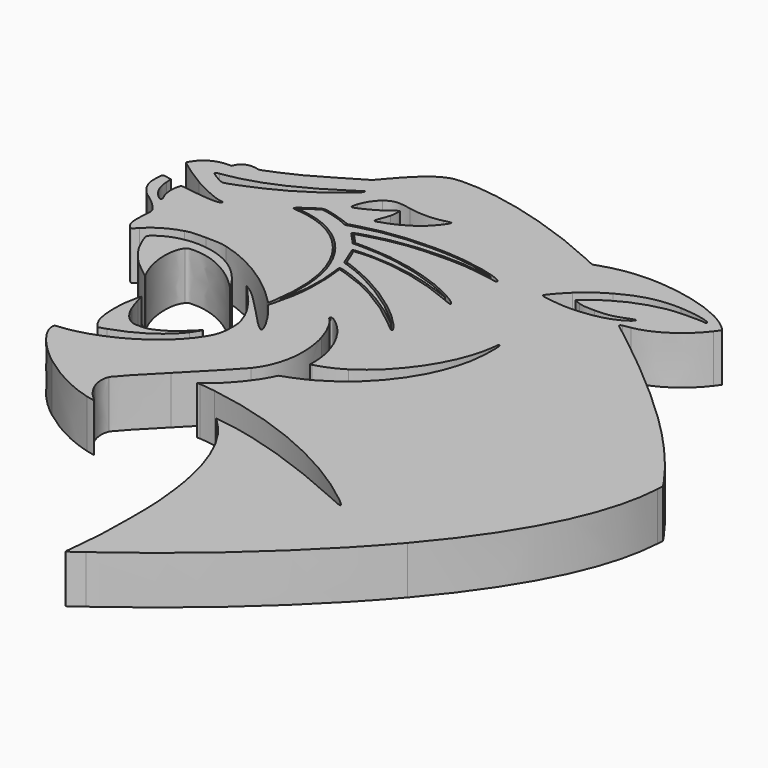
from build123d import *

# Parameters (mm, degrees)
F1_DEPTH = 10


# Not quite as in the source:
# - ends of sketch curves that miss each other by under 0.0002 mm in the source are joined


with BuildPart() as f1:
    # F0 (on Top) → F1 (new body)
    with BuildSketch(Plane.XY):
        with BuildLine():
            add(Edge.make_bspline(
                [(-23.607011, 20.41253), (-23.555899, 20.466755), (-23.36464, 21.326937), (-23.181995, 22.324017)],
                knots=[0, 0, 0, 0, 1, 1, 1, 1], degree=3))
            add(Edge.make_bspline(
                [(-23.181995, 22.324017), (-22.492284, 26.088964), (-22.389352, 30.089862), (-22.897956, 33.36236)],
                knots=[0, 0, 0, 0, 1, 1, 1, 1], degree=3))
            add(Edge.make_bspline(
                [(-22.897956, 33.36236), (-23.019357, 34.143477), (-23.068107, 34.840872), (-23.006291, 34.912122)],
                knots=[0, 0, 0, 0, 1, 1, 1, 1], degree=3))
            add(Edge.make_bspline(
                [(-23.006291, 34.912122), (-22.769167, 35.185415), (-18.48955, 33.680779), (-15.558898, 32.29376)],
                knots=[0, 0, 0, 0, 1, 1, 1, 1], degree=3))
            add(Edge.make_bspline(
                [(-15.558898, 32.29376), (-12.058682, 30.637175), (-7.348256, 27.560307), (-4.801806, 25.267182)],
                knots=[0, 0, 0, 0, 1, 1, 1, 1], degree=3))
            add(Edge.make_bspline(
                [(-4.801806, 25.267182), (-4.500624, 24.995967), (-4.300395, 24.860352), (-4.356852, 24.96584)],
                knots=[0, 0, 0, 0, 1, 1, 1, 1], degree=3))
            add(Edge.make_bspline(
                [(-4.356852, 24.96584), (-4.574715, 25.372872), (-7.364497, 27.840845), (-9.01195, 29.083962)],
                knots=[0, 0, 0, 0, 1, 1, 1, 1], degree=3))
            add(Edge.make_bspline(
                [(-9.01195, 29.083962), (-13.459709, 32.440107), (-18.866425, 35.386422), (-22.748893, 36.569729)],
                knots=[0, 0, 0, 0, 1, 1, 1, 1], degree=3))
            add(Edge.make_bspline(
                [(-22.748893, 36.569729), (-23.476911, 36.791617), (-23.718841, 36.937543), (-23.775043, 37.188685)],
                knots=[0, 0, 0, 0, 1, 1, 1, 1], degree=3))
            add(Edge.make_bspline(
                [(-23.775043, 37.188685), (-23.81549, 37.369424), (-24.179792, 38.281077), (-24.584599, 39.214579)],
                knots=[0, 0, 0, 0, 1, 1, 1, 1], degree=3))
            add(Edge.make_bspline(
                [(-24.584599, 39.214579), (-24.989408, 40.148082), (-25.320615, 40.980952), (-25.320615, 41.065402)],
                knots=[0, 0, 0, 0, 1, 1, 1, 1], degree=3))
            add(Edge.make_bspline(
                [(-25.320615, 41.065402), (-25.320615, 41.330584), (-24.374488, 41.416412), (-21.450763, 41.416462)],
                knots=[0, 0, 0, 0, 1, 1, 1, 1], degree=3))
            add(Edge.make_bspline(
                [(-21.450763, 41.416462), (-15.907912, 41.416555), (-10.712137, 40.427282), (-5.242939, 38.3305)],
                knots=[0, 0, 0, 0, 1, 1, 1, 1], degree=3))
            add(Edge.make_bspline(
                [(-5.242939, 38.3305), (-4.044155, 37.87091), (-3.111244, 37.541015), (-3.169804, 37.597399)],
                knots=[0, 0, 0, 0, 1, 1, 1, 1], degree=3))
            add(Edge.make_bspline(
                [(-3.169804, 37.597399), (-3.452747, 37.869826), (-5.755507, 38.953568), (-7.588494, 39.676957)],
                knots=[0, 0, 0, 0, 1, 1, 1, 1], degree=3))
            add(Edge.make_bspline(
                [(-7.588494, 39.676957), (-13.021844, 41.821228), (-19.037966, 43.012825), (-24.43056, 43.012825)],
                knots=[0, 0, 0, 0, 1, 1, 1, 1], degree=3))
            Line((-24.43056, 43.012825), (-26.740849, 43.012825))
            Line((-26.740849, 43.012825), (-27.585583, 43.951994))
            add(Edge.make_bspline(
                [(-27.585583, 43.951994), (-28.050187, 44.468535), (-28.6169, 45.072836), (-28.844945, 45.294882)],
                knots=[0, 0, 0, 0, 1, 1, 1, 1], degree=3))
            add(Edge.make_bspline(
                [(-28.844945, 45.294882), (-29.131999, 45.574386), (-29.215641, 45.750195), (-29.11679, 45.866281)],
                knots=[0, 0, 0, 0, 1, 1, 1, 1], degree=3))
            add(Edge.make_bspline(
                [(-29.11679, 45.866281), (-28.899874, 46.121018), (-24.878314, 47.26273), (-22.658669, 47.699727)],
                knots=[0, 0, 0, 0, 1, 1, 1, 1], degree=3))
            add(Edge.make_bspline(
                [(-22.658669, 47.699727), (-16.690853, 48.874652), (-10.13353, 49.022795), (-4.036425, 48.120442)],
                knots=[0, 0, 0, 0, 1, 1, 1, 1], degree=3))
            add(Edge.make_bspline(
                [(-4.036425, 48.120442), (-2.934208, 47.957317), (-2.012859, 47.845072), (-1.988982, 47.871005)],
                knots=[0, 0, 0, 0, 1, 1, 1, 1], degree=3))
            add(Edge.make_bspline(
                [(-1.988982, 47.871005), (-1.885069, 47.983876), (-5.101598, 48.762421), (-6.86971, 49.052363)],
                knots=[0, 0, 0, 0, 1, 1, 1, 1], degree=3))
            add(Edge.make_bspline(
                [(-6.86971, 49.052363), (-9.744468, 49.523776), (-12.162409, 49.703075), (-15.639058, 49.702643)],
                knots=[0, 0, 0, 0, 1, 1, 1, 1], degree=3))
            add(Edge.make_bspline(
                [(-15.639058, 49.702643), (-21.335491, 49.701981), (-25.526134, 49.145658), (-30.173319, 47.773322)],
                knots=[0, 0, 0, 0, 1, 1, 1, 1], degree=3))
            Line((-30.173319, 47.773322), (-31.778112, 47.299418))
            Line((-31.778112, 47.299418), (-32.799291, 47.76548))
            add(Edge.make_bspline(
                [(-32.799291, 47.76548), (-33.932578, 48.282708), (-35.678107, 48.809259), (-37.107958, 49.06522)],
                knots=[0, 0, 0, 0, 1, 1, 1, 1], degree=3))
            Line((-37.107958, 49.06522), (-38.045893, 49.233122))
            Line((-38.045893, 49.233122), (-39.730176, 48.074284))
            Line((-39.730176, 48.074284), (-41.414458, 46.915445))
            Line((-41.414458, 46.915445), (-40.865376, 46.87577))
            add(Edge.make_bspline(
                [(-40.865376, 46.87577), (-32.764973, 46.290472), (-26.281806, 40.581082), (-24.167065, 32.17043)],
                knots=[0, 0, 0, 0, 1, 1, 1, 1], degree=3))
            add(Edge.make_bspline(
                [(-24.167065, 32.17043), (-23.525104, 29.617257), (-23.341412, 27.648612), (-23.432327, 24.296187)],
                knots=[0, 0, 0, 0, 1, 1, 1, 1], degree=3))
            add(Edge.make_bspline(
                [(-23.432327, 24.296187), (-23.47747, 22.6316), (-23.556139, 21.054619), (-23.607149, 20.79179)],
                knots=[0, 0, 0, 0, 1, 1, 1, 1], degree=3))
            add(Edge.make_bspline(
                [(-23.607149, 20.79179), (-23.658157, 20.52896), (-23.658074, 20.358297), (-23.607011, 20.41253)],
                knots=[0, 0, 0, 0, 1, 1, 1, 1], degree=3))
        make_face()
    extrude(amount=F1_DEPTH)


with BuildPart() as f1b:
    # F0 (on Top) → F1, piece 2 (new body)
    with BuildSketch(Plane.XY):
        with BuildLine():
            add(Edge.make_bspline(
                [(4.705259, -70.782003), (4.800284, -70.717803), (5.966422, -69.878711), (7.296682, -68.917368)],
                knots=[0, 0, 0, 0, 1, 1, 1, 1], degree=3))
            add(Edge.make_bspline(
                [(7.296682, -68.917368), (21.832102, -58.413018), (35.938987, -45.615086), (46.067909, -33.743658)],
                knots=[0, 0, 0, 0, 1, 1, 1, 1], degree=3))
            add(Edge.make_bspline(
                [(46.067909, -33.743658), (58.546252, -19.118643), (65.216864, -5.670423), (65.968147, 6.375994)],
                knots=[0, 0, 0, 0, 1, 1, 1, 1], degree=3))
            Line((65.968147, 6.375994), (66.052589, 7.729962))
            Line((66.052589, 7.729962), (65.261452, 8.924637))
            add(Edge.make_bspline(
                [(65.261452, 8.924637), (62.172787, 13.588767), (56.377229, 20.249052), (50.267025, 26.156322)],
                knots=[0, 0, 0, 0, 1, 1, 1, 1], degree=3))
            add(Edge.make_bspline(
                [(50.267025, 26.156322), (44.572132, 31.662079), (36.743707, 38.382701), (28.749952, 44.628517)],
                knots=[0, 0, 0, 0, 1, 1, 1, 1], degree=3))
            add(Edge.make_bspline(
                [(28.749952, 44.628517), (26.946637, 46.03751), (25.393462, 47.225745), (25.298437, 47.269039)],
                knots=[0, 0, 0, 0, 1, 1, 1, 1], degree=3))
            add(Edge.make_bspline(
                [(25.298437, 47.269039), (24.962047, 47.422312), (25.129792, 47.777819), (25.574857, 47.854874)],
                knots=[0, 0, 0, 0, 1, 1, 1, 1], degree=3))
            add(Edge.make_bspline(
                [(25.574857, 47.854874), (25.821907, 47.897639), (26.52159, 48.014086), (27.129712, 48.11363)],
                knots=[0, 0, 0, 0, 1, 1, 1, 1], degree=3))
            add(Edge.make_bspline(
                [(27.129712, 48.11363), (30.990434, 48.7456), (35.53944, 51.72252), (38.360805, 55.46339)],
                knots=[0, 0, 0, 0, 1, 1, 1, 1], degree=3))
            Line((38.360805, 55.46339), (39.226222, 56.610857))
            Line((39.226222, 56.610857), (38.845079, 57.069367))
            add(Edge.make_bspline(
                [(38.845079, 57.069367), (38.271149, 57.759803), (36.417944, 59.076346), (35.075152, 59.747583)],
                knots=[0, 0, 0, 0, 1, 1, 1, 1], degree=3))
            add(Edge.make_bspline(
                [(35.075152, 59.747583), (29.657917, 62.455558), (21.886829, 63.858181), (15.727462, 63.239696)],
                knots=[0, 0, 0, 0, 1, 1, 1, 1], degree=3))
            add(Edge.make_bspline(
                [(15.727462, 63.239696), (13.626052, 63.028686), (11.416064, 62.566846), (9.706604, 61.981468)],
                knots=[0, 0, 0, 0, 1, 1, 1, 1], degree=3))
            Line((9.706604, 61.981468), (8.315737, 61.505189))
            Line((8.315737, 61.505189), (6.251369, 62.462768))
            add(Edge.make_bspline(
                [(6.251369, 62.462768), (-2.233126, 66.398401), (-11.305424, 69.319675), (-18.893895, 70.559529)],
                knots=[0, 0, 0, 0, 1, 1, 1, 1], degree=3))
            add(Edge.make_bspline(
                [(-18.893895, 70.559529), (-23.141778, 71.253575), (-27.035465, 71.358933), (-28.706736, 70.82505)],
                knots=[0, 0, 0, 0, 1, 1, 1, 1], degree=3))
            add(Edge.make_bspline(
                [(-28.706736, 70.82505), (-30.890658, 70.127402), (-33.141897, 68.280899), (-36.351063, 64.555048)],
                knots=[0, 0, 0, 0, 1, 1, 1, 1], degree=3))
            Line((-36.351063, 64.555048), (-38.19061, 62.419328))
            Line((-38.19061, 62.419328), (-43.261514, 59.416793))
            add(Edge.make_bspline(
                [(-43.261514, 59.416793), (-47.604785, 56.845096), (-48.792569, 56.217863), (-51.539241, 55.045585)],
                knots=[0, 0, 0, 0, 1, 1, 1, 1], degree=3))
            add(Edge.make_bspline(
                [(-51.539241, 55.045585), (-54.681867, 53.704314), (-54.758811, 53.680613), (-55.382683, 53.861668)],
                knots=[0, 0, 0, 0, 1, 1, 1, 1], degree=3))
            add(Edge.make_bspline(
                [(-55.382683, 53.861668), (-56.252499, 54.114099), (-57.539176, 53.957718), (-58.145414, 53.525892)],
                knots=[0, 0, 0, 0, 1, 1, 1, 1], degree=3))
            add(Edge.make_bspline(
                [(-58.145414, 53.525892), (-58.415377, 53.333596), (-58.751815, 52.916657), (-58.893055, 52.59936)],
                knots=[0, 0, 0, 0, 1, 1, 1, 1], degree=3))
            Line((-58.893055, 52.59936), (-59.149853, 52.022457))
            Line((-59.149853, 52.022457), (-60.250538, 51.98762))
            add(Edge.make_bspline(
                [(-60.250538, 51.98762), (-62.216213, 51.925392), (-64.016752, 50.950571), (-65.122573, 49.349873)],
                knots=[0, 0, 0, 0, 1, 1, 1, 1], degree=3))
            add(Edge.make_bspline(
                [(-65.122573, 49.349873), (-65.427865, 48.907955), (-65.67765, 48.463667), (-65.67765, 48.362565)],
                knots=[0, 0, 0, 0, 1, 1, 1, 1], degree=3))
            add(Edge.make_bspline(
                [(-65.67765, 48.362565), (-65.67765, 48.134593), (-61.718886, 45.422231), (-59.665558, 44.243358)],
                knots=[0, 0, 0, 0, 1, 1, 1, 1], degree=3))
            add(Edge.make_bspline(
                [(-59.665558, 44.243358), (-56.74652, 42.567457), (-53.65725, 41.262505), (-52.60538, 41.261037)],
                knots=[0, 0, 0, 0, 1, 1, 1, 1], degree=3))
            add(Edge.make_bspline(
                [(-52.60538, 41.261037), (-52.444907, 41.260878), (-52.317444, 41.157422), (-52.317444, 41.027479)],
                knots=[0, 0, 0, 0, 1, 1, 1, 1], degree=3))
            add(Edge.make_bspline(
                [(-52.317444, 41.027479), (-52.317444, 40.518796), (-54.934684, 40.524318), (-58.283467, 41.040064)],
                knots=[0, 0, 0, 0, 1, 1, 1, 1], degree=3))
            add(Edge.make_bspline(
                [(-58.283467, 41.040064), (-61.427327, 41.524253), (-61.066151, 41.547586), (-61.326406, 40.843484)],
                knots=[0, 0, 0, 0, 1, 1, 1, 1], degree=3))
            add(Edge.make_bspline(
                [(-61.326406, 40.843484), (-61.682848, 39.879152), (-61.555269, 37.882482), (-61.073767, 36.889573)],
                knots=[0, 0, 0, 0, 1, 1, 1, 1], degree=3))
            add(Edge.make_bspline(
                [(-61.073767, 36.889573), (-60.450511, 35.604357), (-60.651031, 35.33126), (-61.622458, 36.142298)],
                knots=[0, 0, 0, 0, 1, 1, 1, 1], degree=3))
            add(Edge.make_bspline(
                [(-61.622458, 36.142298), (-62.994686, 37.287958), (-63.731364, 38.882436), (-63.846671, 40.956425)],
                knots=[0, 0, 0, 0, 1, 1, 1, 1], degree=3))
            Line((-63.846671, 40.956425), (-63.913894, 42.165479))
            Line((-63.913894, 42.165479), (-64.806318, 42.369922))
            add(Edge.make_bspline(
                [(-64.806318, 42.369922), (-65.489317, 42.526394), (-65.73681, 42.530496), (-65.860958, 42.387412)],
                knots=[0, 0, 0, 0, 1, 1, 1, 1], degree=3))
            add(Edge.make_bspline(
                [(-65.860958, 42.387412), (-65.961651, 42.27136), (-66.023174, 41.643375), (-66.023174, 40.731629)],
                knots=[0, 0, 0, 0, 1, 1, 1, 1], degree=3))
            add(Edge.make_bspline(
                [(-66.023174, 40.731629), (-66.023174, 39.393592), (-65.982802, 39.168292), (-65.569769, 38.201327)],
                knots=[0, 0, 0, 0, 1, 1, 1, 1], degree=3))
            add(Edge.make_bspline(
                [(-65.569769, 38.201327), (-65.104816, 37.11281), (-64.108529, 35.907057), (-63.267654, 35.415185)],
                knots=[0, 0, 0, 0, 1, 1, 1, 1], degree=3))
            add(Edge.make_bspline(
                [(-63.267654, 35.415185), (-62.599269, 35.024217), (-61.110235, 33.773224), (-60.379088, 32.988394)],
                knots=[0, 0, 0, 0, 1, 1, 1, 1], degree=3))
            add(Edge.make_bspline(
                [(-60.379088, 32.988394), (-59.327598, 31.859704), (-59.272552, 31.657647), (-59.459903, 29.614347)],
                knots=[0, 0, 0, 0, 1, 1, 1, 1], degree=3))
            add(Edge.make_bspline(
                [(-59.459903, 29.614347), (-59.685979, 27.148715), (-59.473531, 25.802075), (-58.747371, 25.097855)],
                knots=[0, 0, 0, 0, 1, 1, 1, 1], degree=3))
            add(Edge.make_bspline(
                [(-58.747371, 25.097855), (-58.518568, 24.875967), (-58.255652, 24.694415), (-58.163113, 24.694415)],
                knots=[0, 0, 0, 0, 1, 1, 1, 1], degree=3))
            add(Edge.make_bspline(
                [(-58.163113, 24.694415), (-58.070574, 24.694415), (-57.624439, 25.092102), (-57.171701, 25.578162)],
                knots=[0, 0, 0, 0, 1, 1, 1, 1], degree=3))
            add(Edge.make_bspline(
                [(-57.171701, 25.578162), (-55.577338, 27.289864), (-53.361754, 28.603219), (-50.813516, 29.347175)],
                knots=[0, 0, 0, 0, 1, 1, 1, 1], degree=3))
            add(Edge.make_bspline(
                [(-50.813516, 29.347175), (-49.715774, 29.667657), (-49.24132, 29.70812), (-46.604806, 29.706109)],
                knots=[0, 0, 0, 0, 1, 1, 1, 1], degree=3))
            add(Edge.make_bspline(
                [(-46.604806, 29.706109), (-44.035113, 29.703859), (-43.437085, 29.65481), (-42.182118, 29.341272)],
                knots=[0, 0, 0, 0, 1, 1, 1, 1], degree=3))
            add(Edge.make_bspline(
                [(-42.182118, 29.341272), (-36.748801, 27.983765), (-30.573919, 24.234147), (-25.639972, 19.296252)],
                knots=[0, 0, 0, 0, 1, 1, 1, 1], degree=3))
            add(Edge.make_bspline(
                [(-25.639972, 19.296252), (-25.017458, 18.673235), (-24.479722, 18.163505), (-24.445, 18.163505)],
                knots=[0, 0, 0, 0, 1, 1, 1, 1], degree=3))
            add(Edge.make_bspline(
                [(-24.445, 18.163505), (-24.410275, 18.163505), (-24.284163, 18.790707), (-24.164742, 19.557297)],
                knots=[0, 0, 0, 0, 1, 1, 1, 1], degree=3))
            add(Edge.make_bspline(
                [(-24.164742, 19.557297), (-22.859161, 27.938074), (-24.328941, 34.930699), (-28.45984, 39.991674)],
                knots=[0, 0, 0, 0, 1, 1, 1, 1], degree=3))
            add(Edge.make_bspline(
                [(-28.45984, 39.991674), (-31.580799, 43.815317), (-35.761267, 45.997984), (-40.83458, 46.452657)],
                knots=[0, 0, 0, 0, 1, 1, 1, 1], degree=3))
            add(Edge.make_bspline(
                [(-40.83458, 46.452657), (-41.658155, 46.526464), (-42.043908, 46.624405), (-42.043908, 46.759696)],
                knots=[0, 0, 0, 0, 1, 1, 1, 1], degree=3))
            add(Edge.make_bspline(
                [(-42.043908, 46.759696), (-42.043908, 46.868956), (-41.212366, 47.540067), (-40.196035, 48.251051)],
                knots=[0, 0, 0, 0, 1, 1, 1, 1], degree=3))
            add(Edge.make_bspline(
                [(-40.196035, 48.251051), (-38.760101, 49.25557), (-38.23346, 49.543748), (-37.83364, 49.543748)],
                knots=[0, 0, 0, 0, 1, 1, 1, 1], degree=3))
            add(Edge.make_bspline(
                [(-37.83364, 49.543748), (-37.00825, 49.543748), (-34.629462, 48.936631), (-33.083735, 48.331471)],
                knots=[0, 0, 0, 0, 1, 1, 1, 1], degree=3))
            Line((-33.083735, 48.331471), (-31.655952, 47.772489))
            Line((-31.655952, 47.772489), (-30.043137, 48.253309))
            add(Edge.make_bspline(
                [(-30.043137, 48.253309), (-24.155488, 50.008567), (-16.453518, 50.572515), (-9.215461, 49.778338)],
                knots=[0, 0, 0, 0, 1, 1, 1, 1], degree=3))
            add(Edge.make_bspline(
                [(-9.215461, 49.778338), (-4.556375, 49.267133), (-0.028366, 48.006765), (-0.028366, 47.221117)],
                knots=[0, 0, 0, 0, 1, 1, 1, 1], degree=3))
            add(Edge.make_bspline(
                [(-0.028366, 47.221117), (-0.028366, 47.025338), (-0.108002, 46.983049), (-0.339336, 47.055988)],
                knots=[0, 0, 0, 0, 1, 1, 1, 1], degree=3))
            add(Edge.make_bspline(
                [(-0.339336, 47.055988), (-1.021156, 47.270956), (-5.468729, 47.942132), (-7.398157, 48.121222)],
                knots=[0, 0, 0, 0, 1, 1, 1, 1], degree=3))
            add(Edge.make_bspline(
                [(-7.398157, 48.121222), (-10.021639, 48.364733), (-16.854103, 48.224521), (-19.239421, 47.878222)],
                knots=[0, 0, 0, 0, 1, 1, 1, 1], degree=3))
            add(Edge.make_bspline(
                [(-19.239421, 47.878222), (-22.390204, 47.420791), (-24.929726, 46.860148), (-27.354446, 46.086689)],
                knots=[0, 0, 0, 0, 1, 1, 1, 1], degree=3))
            Line((-27.354446, 46.086689), (-28.628125, 45.680398))
            Line((-28.628125, 45.680398), (-27.573977, 44.545729))
            Line((-27.573977, 44.545729), (-26.519829, 43.411061))
            Line((-26.519829, 43.411061), (-23.812535, 43.384751))
            add(Edge.make_bspline(
                [(-23.812535, 43.384751), (-18.533455, 43.333459), (-12.836811, 42.177951), (-7.353444, 40.046194)],
                knots=[0, 0, 0, 0, 1, 1, 1, 1], degree=3))
            add(Edge.make_bspline(
                [(-7.353444, 40.046194), (-3.864717, 38.68989), (-0.607285, 36.717341), (-1.037471, 36.221537)],
                knots=[0, 0, 0, 0, 1, 1, 1, 1], degree=3))
            add(Edge.make_bspline(
                [(-1.037471, 36.221537), (-1.079156, 36.173492), (-1.973105, 36.510246), (-3.024025, 36.969877)],
                knots=[0, 0, 0, 0, 1, 1, 1, 1], degree=3))
            add(Edge.make_bspline(
                [(-3.024025, 36.969877), (-9.987491, 40.015423), (-18.305543, 41.61443), (-23.974898, 40.997338)],
                knots=[0, 0, 0, 0, 1, 1, 1, 1], degree=3))
            Line((-23.974898, 40.997338), (-24.909626, 40.895593))
            Line((-24.909626, 40.895593), (-24.517787, 40.082549))
            add(Edge.make_bspline(
                [(-24.517787, 40.082549), (-24.302274, 39.635375), (-23.95006, 38.785657), (-23.735085, 38.194291)],
                knots=[0, 0, 0, 0, 1, 1, 1, 1], degree=3))
            add(Edge.make_bspline(
                [(-23.735085, 38.194291), (-23.48472, 37.50557), (-23.264736, 37.118425), (-23.123091, 37.117261)],
                knots=[0, 0, 0, 0, 1, 1, 1, 1], degree=3))
            add(Edge.make_bspline(
                [(-23.123091, 37.117261), (-22.679019, 37.113586), (-18.842861, 35.537127), (-16.965657, 34.586839)],
                knots=[0, 0, 0, 0, 1, 1, 1, 1], degree=3))
            add(Edge.make_bspline(
                [(-16.965657, 34.586839), (-11.909682, 32.027397), (-6.676796, 28.194139), (-3.863666, 24.989209)],
                knots=[0, 0, 0, 0, 1, 1, 1, 1], degree=3))
            add(Edge.make_bspline(
                [(-3.863666, 24.989209), (-2.764372, 23.736815), (-2.406964, 23.101512), (-2.801682, 23.101512)],
                knots=[0, 0, 0, 0, 1, 1, 1, 1], degree=3))
            add(Edge.make_bspline(
                [(-2.801682, 23.101512), (-2.882722, 23.101512), (-3.768988, 23.809257), (-4.771161, 24.674284)],
                knots=[0, 0, 0, 0, 1, 1, 1, 1], degree=3))
            add(Edge.make_bspline(
                [(-4.771161, 24.674284), (-9.785466, 29.002362), (-15.67434, 32.380272), (-21.15676, 34.073202)],
                knots=[0, 0, 0, 0, 1, 1, 1, 1], degree=3))
            Line((-21.15676, 34.073202), (-22.727057, 34.558099))
            Line((-22.727057, 34.558099), (-22.650259, 34.115532))
            add(Edge.make_bspline(
                [(-22.650259, 34.115532), (-22.129136, 31.112472), (-22.177762, 25.842454), (-22.756295, 22.623642)],
                knots=[0, 0, 0, 0, 1, 1, 1, 1], degree=3))
            add(Edge.make_bspline(
                [(-22.756295, 22.623642), (-22.953128, 21.528514), (-23.306635, 19.932094), (-23.541868, 19.076022)],
                knots=[0, 0, 0, 0, 1, 1, 1, 1], degree=3))
            Line((-23.541868, 19.076022), (-23.969566, 17.51954))
            Line((-23.969566, 17.51954), (-22.950735, 16.288437))
            add(Edge.make_bspline(
                [(-22.950735, 16.288437), (-21.324874, 14.323834), (-19.648169, 11.604762), (-19.367809, 10.478089)],
                knots=[0, 0, 0, 0, 1, 1, 1, 1], degree=3))
            add(Edge.make_bspline(
                [(-19.367809, 10.478089), (-19.084441, 9.339335), (-20.25021, 10.327459), (-24.169221, 14.547852)],
                knots=[0, 0, 0, 0, 1, 1, 1, 1], degree=3))
            add(Edge.make_bspline(
                [(-24.169221, 14.547852), (-27.041818, 17.641362), (-28.867624, 19.356312), (-30.063521, 20.084284)],
                knots=[0, 0, 0, 0, 1, 1, 1, 1], degree=3))
            Line((-30.063521, 20.084284), (-30.918082, 20.60447))
            Line((-30.918082, 20.60447), (-29.881515, 19.512042))
            add(Edge.make_bspline(
                [(-29.881515, 19.512042), (-26.667872, 16.125214), (-24.911653, 13.48775), (-23.998393, 10.676847)],
                knots=[0, 0, 0, 0, 1, 1, 1, 1], degree=3))
            add(Edge.make_bspline(
                [(-23.998393, 10.676847), (-23.66262, 9.643377), (-23.60908, 9.24572), (-23.601624, 7.72997)],
                knots=[0, 0, 0, 0, 1, 1, 1, 1], degree=3))
            add(Edge.make_bspline(
                [(-23.601624, 7.72997), (-23.591199, 5.611385), (-23.908683, 4.364892), (-24.873884, 2.73482)],
                knots=[0, 0, 0, 0, 1, 1, 1, 1], degree=3))
            add(Edge.make_bspline(
                [(-24.873884, 2.73482), (-28.649692, -3.641928), (-37.895355, -9.093655), (-46.051971, -9.752898)],
                knots=[0, 0, 0, 0, 1, 1, 1, 1], degree=3))
            add(Edge.make_bspline(
                [(-46.051971, -9.752898), (-46.448839, -9.784998), (-46.544303, -9.862241), (-46.583598, -10.183218)],
                knots=[0, 0, 0, 0, 1, 1, 1, 1], degree=3))
            add(Edge.make_bspline(
                [(-46.583598, -10.183218), (-46.824929, -12.154435), (-43.604748, -16.272881), (-39.129191, -19.717023)],
                knots=[0, 0, 0, 0, 1, 1, 1, 1], degree=3))
            add(Edge.make_bspline(
                [(-39.129191, -19.717023), (-35.215469, -22.728813), (-30.904956, -24.938013), (-26.798638, -26.036605)],
                knots=[0, 0, 0, 0, 1, 1, 1, 1], degree=3))
            add(Edge.make_bspline(
                [(-26.798638, -26.036605), (-25.901212, -26.276703), (-25.137249, -26.438913), (-25.100942, -26.397063)],
                knots=[0, 0, 0, 0, 1, 1, 1, 1], degree=3))
            add(Edge.make_bspline(
                [(-25.100942, -26.397063), (-25.064634, -26.355213), (-25.352577, -26.042635), (-25.740811, -25.702435)],
                knots=[0, 0, 0, 0, 1, 1, 1, 1], degree=3))
            add(Edge.make_bspline(
                [(-25.740811, -25.702435), (-26.69118, -24.869651), (-27.619091, -23.551788), (-28.139085, -22.296303)],
                knots=[0, 0, 0, 0, 1, 1, 1, 1], degree=3))
            add(Edge.make_bspline(
                [(-28.139085, -22.296303), (-28.700998, -20.939606), (-28.746615, -19.360938), (-28.250477, -18.441318)],
                knots=[0, 0, 0, 0, 1, 1, 1, 1], degree=3))
            add(Edge.make_bspline(
                [(-28.250477, -18.441318), (-27.881832, -17.758023), (-25.904229, -15.637518), (-21.324419, -11.01478)],
                knots=[0, 0, 0, 0, 1, 1, 1, 1], degree=3))
            add(Edge.make_bspline(
                [(-21.324419, -11.01478), (-16.83985, -6.488178), (-12.922369, -2.409228), (-12.255099, -1.571643)],
                knots=[0, 0, 0, 0, 1, 1, 1, 1], degree=3))
            add(Edge.make_bspline(
                [(-12.255099, -1.571643), (-9.177396, 2.291622), (-8.337201, 8.067814), (-9.99957, 13.934697)],
                knots=[0, 0, 0, 0, 1, 1, 1, 1], degree=3))
            add(Edge.make_bspline(
                [(-9.99957, 13.934697), (-10.659027, 16.262067), (-12.014752, 18.881442), (-13.038081, 19.805352)],
                knots=[0, 0, 0, 0, 1, 1, 1, 1], degree=3))
            add(Edge.make_bspline(
                [(-13.038081, 19.805352), (-13.325145, 20.064529), (-13.391434, 20.216277), (-13.295044, 20.393569)],
                knots=[0, 0, 0, 0, 1, 1, 1, 1], degree=3))
            add(Edge.make_bspline(
                [(-13.295044, 20.393569), (-12.988371, 20.957659), (-10.485909, 18.885897), (-8.983326, 16.823937)],
                knots=[0, 0, 0, 0, 1, 1, 1, 1], degree=3))
            add(Edge.make_bspline(
                [(-8.983326, 16.823937), (-6.88978, 13.951017), (-5.563471, 10.011642), (-5.558542, 6.651724)],
                knots=[0, 0, 0, 0, 1, 1, 1, 1], degree=3))
            Line((-5.558542, 6.651724), (-5.556742, 5.414187))
            Line((-5.556742, 5.414187), (-5.176667, 5.512054))
            add(Edge.make_bspline(
                [(-5.176667, 5.512054), (-3.198481, 6.021424), (-1.351209, 6.831987), (0.45535, 7.983312)],
                knots=[0, 0, 0, 0, 1, 1, 1, 1], degree=3))
            add(Edge.make_bspline(
                [(0.45535, 7.983312), (7.221637, 12.295489), (12.80283, 20.715574), (13.855049, 28.198812)],
                knots=[0, 0, 0, 0, 1, 1, 1, 1], degree=3))
            add(Edge.make_bspline(
                [(13.855049, 28.198812), (13.972072, 29.031102), (14.068079, 29.765832), (14.06838, 29.831539)],
                knots=[0, 0, 0, 0, 1, 1, 1, 1], degree=3))
            add(Edge.make_bspline(
                [(14.06838, 29.831539), (14.068657, 29.897239), (14.153054, 29.951007), (14.255864, 29.951007)],
                knots=[0, 0, 0, 0, 1, 1, 1, 1], degree=3))
            add(Edge.make_bspline(
                [(14.255864, 29.951007), (14.707612, 29.951007), (14.635882, 25.505165), (14.139449, 22.735489)],
                knots=[0, 0, 0, 0, 1, 1, 1, 1], degree=3))
            add(Edge.make_bspline(
                [(14.139449, 22.735489), (13.697639, 20.270585), (12.583807, 17.048584), (11.374995, 14.738757)],
                knots=[0, 0, 0, 0, 1, 1, 1, 1], degree=3))
            add(Edge.make_bspline(
                [(11.374995, 14.738757), (7.803322, 7.9139), (1.780057, 2.460012), (-5.04592, -0.129903)],
                knots=[0, 0, 0, 0, 1, 1, 1, 1], degree=3))
            Line((-5.04592, -0.129903), (-7.091964, -0.906206))
            Line((-7.091964, -0.906206), (-7.645663, -1.998258))
            add(Edge.make_bspline(
                [(-7.645663, -1.998258), (-9.153951, -4.973028), (-12.423561, -8.776931), (-15.022665, -10.580763)],
                knots=[0, 0, 0, 0, 1, 1, 1, 1], degree=3))
            Line((-15.022665, -10.580763), (-15.837047, -11.145963))
            Line((-15.837047, -11.145963), (-15.192854, -11.145963))
            add(Edge.make_bspline(
                [(-15.192854, -11.145963), (-14.838548, -11.145963), (-13.349549, -11.321913), (-11.883968, -11.536961)],
                knots=[0, 0, 0, 0, 1, 1, 1, 1], degree=3))
            add(Edge.make_bspline(
                [(-11.883968, -11.536961), (2.463074, -13.642143), (16.864807, -19.870451), (27.854099, -28.722446)],
                knots=[0, 0, 0, 0, 1, 1, 1, 1], degree=3))
            add(Edge.make_bspline(
                [(27.854099, -28.722446), (29.139067, -29.757506), (29.549782, -30.260831), (29.109434, -30.260831)],
                knots=[0, 0, 0, 0, 1, 1, 1, 1], degree=3))
            add(Edge.make_bspline(
                [(29.109434, -30.260831), (29.020057, -30.260831), (27.542947, -29.622626), (25.826962, -28.842588)],
                knots=[0, 0, 0, 0, 1, 1, 1, 1], degree=3))
            add(Edge.make_bspline(
                [(25.826962, -28.842588), (13.854442, -23.400243), (3.068159, -19.944348), (-4.796587, -19.030908)],
                knots=[0, 0, 0, 0, 1, 1, 1, 1], degree=3))
            Line((-4.796587, -19.030908), (-5.625841, -18.934601))
            Line((-5.625841, -18.934601), (-5.14211, -19.374506))
            add(Edge.make_bspline(
                [(-5.14211, -19.374506), (-4.285963, -20.153096), (-2.650805, -22.028036), (-1.899389, -23.092758)],
                knots=[0, 0, 0, 0, 1, 1, 1, 1], degree=3))
            add(Edge.make_bspline(
                [(-1.899389, -23.092758), (1.422097, -27.799143), (3.640229, -34.264953), (4.729732, -42.416531)],
                knots=[0, 0, 0, 0, 1, 1, 1, 1], degree=3))
            add(Edge.make_bspline(
                [(4.729732, -42.416531), (5.330339, -46.910253), (5.431327, -48.769706), (5.423444, -55.189803)],
                knots=[0, 0, 0, 0, 1, 1, 1, 1], degree=3))
            add(Edge.make_bspline(
                [(5.423444, -55.189803), (5.415944, -61.269056), (5.262682, -64.255511), (4.733159, -68.637768)],
                knots=[0, 0, 0, 0, 1, 1, 1, 1], degree=3))
            add(Edge.make_bspline(
                [(4.733159, -68.637768), (4.484624, -70.694568), (4.481527, -70.933188), (4.705259, -70.782003)],
                knots=[0, 0, 0, 0, 1, 1, 1, 1], degree=3))
        make_face()
        with BuildLine():
            add(Edge.make_bspline(
                [(-56.650833, 46.52536), (-56.864647, 46.529785), (-57.645979, 46.888939), (-58.387125, 47.323363)],
                knots=[0, 0, 0, 0, 1, 1, 1, 1], degree=3))
            add(Edge.make_bspline(
                [(-58.387125, 47.323363), (-59.13617, 47.762419), (-59.734661, 48.213566), (-59.734661, 48.339148)],
                knots=[0, 0, 0, 0, 1, 1, 1, 1], degree=3))
            add(Edge.make_bspline(
                [(-59.734661, 48.339148), (-59.734661, 48.496183), (-59.49234, 48.596129), (-58.93996, 48.666925)],
                knots=[0, 0, 0, 0, 1, 1, 1, 1], degree=3))
            add(Edge.make_bspline(
                [(-58.93996, 48.666925), (-52.877837, 49.443875), (-46.145088, 52.32023), (-38.572072, 57.368459)],
                knots=[0, 0, 0, 0, 1, 1, 1, 1], degree=3))
            add(Edge.make_bspline(
                [(-38.572072, 57.368459), (-37.536736, 58.058624), (-36.660837, 58.623303), (-36.625629, 58.623303)],
                knots=[0, 0, 0, 0, 1, 1, 1, 1], degree=3))
            add(Edge.make_bspline(
                [(-36.625629, 58.623303), (-36.590424, 58.623303), (-36.561616, 58.509354), (-36.561616, 58.370081)],
                knots=[0, 0, 0, 0, 1, 1, 1, 1], degree=3))
            add(Edge.make_bspline(
                [(-36.561616, 58.370081), (-36.561616, 58.230811), (-37.164723, 57.590456), (-37.901853, 56.947072)],
                knots=[0, 0, 0, 0, 1, 1, 1, 1], degree=3))
            add(Edge.make_bspline(
                [(-37.901853, 56.947072), (-42.439229, 52.986746), (-47.999518, 49.697485), (-54.174763, 47.320627)],
                knots=[0, 0, 0, 0, 1, 1, 1, 1], degree=3))
            add(Edge.make_bspline(
                [(-54.174763, 47.320627), (-55.322786, 46.878752), (-56.437018, 46.520882), (-56.650833, 46.52536)],
                knots=[0, 0, 0, 0, 1, 1, 1, 1], degree=3))
        make_face(mode=Mode.SUBTRACT)
        with BuildLine():
            add(Edge.make_bspline(
                [(-26.746954, 52.021816), (-28.673381, 51.293225), (-28.904455, 51.241075), (-28.995444, 51.514357)],
                knots=[0, 0, 0, 0, 1, 1, 1, 1], degree=3))
            add(Edge.make_bspline(
                [(-28.995444, 51.514357), (-29.036879, 51.638797), (-28.887023, 52.160243), (-28.662432, 52.673129)],
                knots=[0, 0, 0, 0, 1, 1, 1, 1], degree=3))
            add(Edge.make_bspline(
                [(-28.662432, 52.673129), (-28.437839, 53.186016), (-28.153799, 53.994985), (-28.031231, 54.470836)],
                knots=[0, 0, 0, 0, 1, 1, 1, 1], degree=3))
            add(Edge.make_bspline(
                [(-28.031231, 54.470836), (-27.793596, 55.393409), (-27.731352, 56.711815), (-27.925431, 56.711815)],
                knots=[0, 0, 0, 0, 1, 1, 1, 1], degree=3))
            add(Edge.make_bspline(
                [(-27.925431, 56.711815), (-27.989811, 56.711815), (-28.565105, 56.306419), (-29.203864, 55.810937)],
                knots=[0, 0, 0, 0, 1, 1, 1, 1], degree=3))
            add(Edge.make_bspline(
                [(-29.203864, 55.810937), (-30.899434, 54.495687), (-33.943983, 52.888841), (-34.740465, 52.888841)],
                knots=[0, 0, 0, 0, 1, 1, 1, 1], degree=3))
            add(Edge.make_bspline(
                [(-34.740465, 52.888841), (-35.063226, 52.888841), (-35.060326, 53.09883), (-34.721902, 54.232495)],
                knots=[0, 0, 0, 0, 1, 1, 1, 1], degree=3))
            add(Edge.make_bspline(
                [(-34.721902, 54.232495), (-34.318833, 55.582741), (-33.354429, 57.043337), (-32.361252, 57.807719)],
                knots=[0, 0, 0, 0, 1, 1, 1, 1], degree=3))
            add(Edge.make_bspline(
                [(-32.361252, 57.807719), (-30.935313, 58.905169), (-30.004782, 59.018042), (-27.201785, 58.433557)],
                knots=[0, 0, 0, 0, 1, 1, 1, 1], degree=3))
            add(Edge.make_bspline(
                [(-27.201785, 58.433557), (-24.789226, 57.930486), (-22.145596, 57.937138), (-20.240473, 58.45107)],
                knots=[0, 0, 0, 0, 1, 1, 1, 1], degree=3))
            add(Edge.make_bspline(
                [(-20.240473, 58.45107), (-19.460796, 58.661399), (-18.78175, 58.786087), (-18.731484, 58.728153)],
                knots=[0, 0, 0, 0, 1, 1, 1, 1], degree=3))
            add(Edge.make_bspline(
                [(-18.731484, 58.728153), (-18.453063, 58.407263), (-20.348721, 56.018931), (-21.884093, 54.756193)],
                knots=[0, 0, 0, 0, 1, 1, 1, 1], degree=3))
            add(Edge.make_bspline(
                [(-21.884093, 54.756193), (-23.084757, 53.76873), (-25.05033, 52.663492), (-26.746954, 52.021816)],
                knots=[0, 0, 0, 0, 1, 1, 1, 1], degree=3))
        make_face(mode=Mode.SUBTRACT)
        with BuildLine():
            add(Edge.make_bspline(
                [(22.683539, 48.436047), (20.108122, 47.451792), (15.949454, 46.991997), (12.548662, 47.315502)],
                knots=[0, 0, 0, 0, 1, 1, 1, 1], degree=3))
            add(Edge.make_bspline(
                [(12.548662, 47.315502), (10.009687, 47.557025), (8.817014, 47.796224), (8.817014, 48.06391)],
                knots=[0, 0, 0, 0, 1, 1, 1, 1], degree=3))
            add(Edge.make_bspline(
                [(8.817014, 48.06391), (8.817014, 48.405333), (10.613414, 50.499472), (11.995822, 51.769569)],
                knots=[0, 0, 0, 0, 1, 1, 1, 1], degree=3))
            add(Edge.make_bspline(
                [(11.995822, 51.769569), (13.787369, 53.415571), (15.340717, 54.554441), (17.316869, 55.670807)],
                knots=[0, 0, 0, 0, 1, 1, 1, 1], degree=3))
            add(Edge.make_bspline(
                [(17.316869, 55.670807), (21.260234, 57.898486), (24.714089, 58.74805), (29.130367, 58.576641)],
                knots=[0, 0, 0, 0, 1, 1, 1, 1], degree=3))
            add(Edge.make_bspline(
                [(29.130367, 58.576641), (32.242492, 58.455851), (35.635964, 57.714091), (35.709247, 57.138601)],
                knots=[0, 0, 0, 0, 1, 1, 1, 1], degree=3))
            add(Edge.make_bspline(
                [(35.709247, 57.138601), (35.739472, 56.900965), (35.672647, 56.878467), (35.237857, 56.979947)],
                knots=[0, 0, 0, 0, 1, 1, 1, 1], degree=3))
            add(Edge.make_bspline(
                [(35.237857, 56.979947), (34.223955, 57.216579), (29.279932, 57.111049), (27.638092, 56.817728)],
                knots=[0, 0, 0, 0, 1, 1, 1, 1], degree=3))
            add(Edge.make_bspline(
                [(27.638092, 56.817728), (24.323917, 56.225637), (21.16653, 55.042083), (18.353437, 53.33735)],
                knots=[0, 0, 0, 0, 1, 1, 1, 1], degree=3))
            add(Edge.make_bspline(
                [(18.353437, 53.33735), (16.575472, 52.259905), (13.875217, 50.181185), (14.02674, 50.006555)],
                knots=[0, 0, 0, 0, 1, 1, 1, 1], degree=3))
            add(Edge.make_bspline(
                [(14.02674, 50.006555), (14.093489, 49.929637), (14.643375, 49.708501), (15.248745, 49.515144)],
                knots=[0, 0, 0, 0, 1, 1, 1, 1], degree=3))
            add(Edge.make_bspline(
                [(15.248745, 49.515144), (16.184092, 49.216385), (16.702289, 49.163437), (18.698962, 49.162603)],
                knots=[0, 0, 0, 0, 1, 1, 1, 1], degree=3))
            add(Edge.make_bspline(
                [(18.698962, 49.162603), (21.260587, 49.161479), (22.393665, 49.384916), (24.828847, 50.371087)],
                knots=[0, 0, 0, 0, 1, 1, 1, 1], degree=3))
            add(Edge.make_bspline(
                [(24.828847, 50.371087), (25.463744, 50.628203), (26.021294, 50.794676), (26.06784, 50.741032)],
                knots=[0, 0, 0, 0, 1, 1, 1, 1], degree=3))
            add(Edge.make_bspline(
                [(26.06784, 50.741032), (26.390069, 50.369647), (24.660232, 49.191488), (22.683539, 48.436047)],
                knots=[0, 0, 0, 0, 1, 1, 1, 1], degree=3))
        make_face(mode=Mode.SUBTRACT)
    extrude(amount=F1_DEPTH)


with BuildPart() as f1c:
    # F0 (on Top) → F1, piece 3 (new body)
    with BuildSketch(Plane.XY):
        with BuildLine():
            add(Edge.make_bspline(
                [(-46.087806, 13.131087), (-46.058128, 13.165287), (-46.220332, 13.576857), (-46.448269, 14.045667)],
                knots=[0, 0, 0, 0, 1, 1, 1, 1], degree=3))
            add(Edge.make_bspline(
                [(-46.448269, 14.045667), (-48.261934, 17.775882), (-48.48085, 22.692875), (-46.917058, 24.574947)],
                knots=[0, 0, 0, 0, 1, 1, 1, 1], degree=3))
            add(Edge.make_bspline(
                [(-46.917058, 24.574947), (-46.570502, 24.992037), (-46.490894, 25.012992), (-45.253119, 25.012992)],
                knots=[0, 0, 0, 0, 1, 1, 1, 1], degree=3))
            add(Edge.make_bspline(
                [(-45.253119, 25.012992), (-41.396867, 25.012992), (-37.163284, 22.935507), (-33.343218, 19.168617)],
                knots=[0, 0, 0, 0, 1, 1, 1, 1], degree=3))
            Line((-33.343218, 19.168617), (-32.727757, 18.561724))
            Line((-32.727757, 18.561724), (-32.997695, 19.093579))
            add(Edge.make_bspline(
                [(-32.997695, 19.093579), (-33.769989, 20.615224), (-35.585137, 22.703284), (-37.294093, 24.03596)],
                knots=[0, 0, 0, 0, 1, 1, 1, 1], degree=3))
            add(Edge.make_bspline(
                [(-37.294093, 24.03596), (-41.737352, 27.500899), (-48.182137, 28.174489), (-52.616897, 25.637449)],
                knots=[0, 0, 0, 0, 1, 1, 1, 1], degree=3))
            add(Edge.make_bspline(
                [(-52.616897, 25.637449), (-53.870119, 24.92051), (-54.483496, 24.363762), (-54.481031, 23.945419)],
                knots=[0, 0, 0, 0, 1, 1, 1, 1], degree=3))
            add(Edge.make_bspline(
                [(-54.481031, 23.945419), (-54.478106, 23.455302), (-53.589074, 21.281187), (-52.910347, 20.104512)],
                knots=[0, 0, 0, 0, 1, 1, 1, 1], degree=3))
            add(Edge.make_bspline(
                [(-52.910347, 20.104512), (-52.116496, 18.728247), (-50.611603, 16.850359), (-49.445583, 15.781009)],
                knots=[0, 0, 0, 0, 1, 1, 1, 1], degree=3))
            add(Edge.make_bspline(
                [(-49.445583, 15.781009), (-48.353077, 14.779077), (-46.159774, 13.048144), (-46.087806, 13.131087)],
                knots=[0, 0, 0, 0, 1, 1, 1, 1], degree=3))
        make_face()
    extrude(amount=F1_DEPTH)


with BuildPart() as f1d:
    # F0 (on Top) → F1, piece 4 (new body)
    with BuildSketch(Plane.XY):
        with BuildLine():
            add(Edge.make_bspline(
                [(-40.654452, -5.889378), (-40.604209, -5.889378), (-39.915938, -5.67556), (-39.124961, -5.414238)],
                knots=[0, 0, 0, 0, 1, 1, 1, 1], degree=3))
            add(Edge.make_bspline(
                [(-39.124961, -5.414238), (-34.266562, -3.809058), (-30.205434, -1.123113), (-27.887592, 2.01794)],
                knots=[0, 0, 0, 0, 1, 1, 1, 1], degree=3))
            add(Edge.make_bspline(
                [(-27.887592, 2.01794), (-27.425942, 2.643552), (-26.927893, 3.3962), (-26.780817, 3.690492)],
                knots=[0, 0, 0, 0, 1, 1, 1, 1], degree=3))
            add(Edge.make_bspline(
                [(-26.780817, 3.690492), (-26.54412, 4.164117), (-26.611008, 4.121952), (-27.363188, 3.323412)],
                knots=[0, 0, 0, 0, 1, 1, 1, 1], degree=3))
            add(Edge.make_bspline(
                [(-27.363188, 3.323412), (-29.224531, 1.347335), (-31.027008, 0.005547), (-32.930055, -0.82066)],
                knots=[0, 0, 0, 0, 1, 1, 1, 1], degree=3))
            add(Edge.make_bspline(
                [(-32.930055, -0.82066), (-33.959489, -1.267578), (-34.26777, -1.328545), (-35.548082, -1.338415)],
                knots=[0, 0, 0, 0, 1, 1, 1, 1], degree=3))
            add(Edge.make_bspline(
                [(-35.548082, -1.338415), (-36.833877, -1.348315), (-37.076258, -1.30429), (-37.674699, -0.952068)],
                knots=[0, 0, 0, 0, 1, 1, 1, 1], degree=3))
            add(Edge.make_bspline(
                [(-37.674699, -0.952068), (-38.802423, -0.288318), (-39.763458, 0.967655), (-40.53072, 2.78045)],
                knots=[0, 0, 0, 0, 1, 1, 1, 1], degree=3))
            add(Edge.make_bspline(
                [(-40.53072, 2.78045), (-40.904205, 3.662877), (-41.33541, 4.952495), (-41.488954, 5.646282)],
                knots=[0, 0, 0, 0, 1, 1, 1, 1], degree=3))
            add(Edge.make_bspline(
                [(-41.488954, 5.646282), (-41.642498, 6.340055), (-41.793325, 6.93674), (-41.824125, 6.972237)],
                knots=[0, 0, 0, 0, 1, 1, 1, 1], degree=3))
            add(Edge.make_bspline(
                [(-41.824125, 6.972237), (-41.854927, 7.007787), (-41.97626, 6.655145), (-42.093759, 6.18869)],
                knots=[0, 0, 0, 0, 1, 1, 1, 1], degree=3))
            add(Edge.make_bspline(
                [(-42.093759, 6.18869), (-42.984032, 2.65448), (-42.930607, -1.806588), (-41.971501, -4.019995)],
                knots=[0, 0, 0, 0, 1, 1, 1, 1], degree=3))
            add(Edge.make_bspline(
                [(-41.971501, -4.019995), (-41.635909, -4.794468), (-40.864503, -5.889378), (-40.654452, -5.889378)],
                knots=[0, 0, 0, 0, 1, 1, 1, 1], degree=3))
        make_face()
    extrude(amount=F1_DEPTH)


solid = Compound([f1.part, f1b.part, f1c.part, f1d.part])
